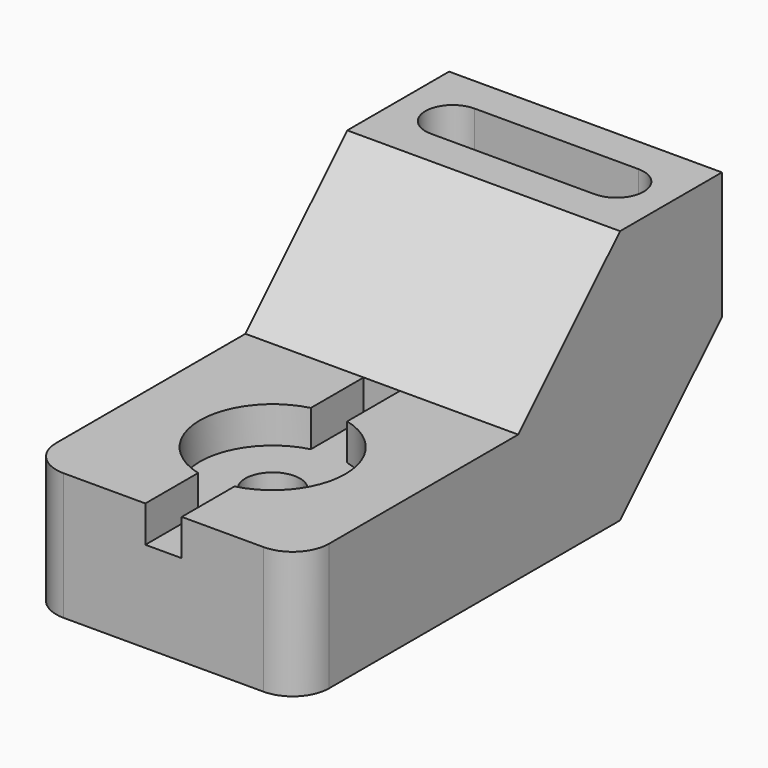
from build123d import *

# Parameters (mm, degrees)
F0_W           = 76.2
F0_H           = 35.56
F1_DEPTH       = 71.12
F0_H_2         = 76.2
F2_DEPTH       = 35.56
F4_DEPTH       = 76.2
F6_D           = 15.24
F6_CBORE_D     = 40.64
F6_CBORE_DEPTH = 10.16
F8_DEPTH       = 27.94
F10_DEPTH      = 10.16
F11_R          = 10.16


with BuildPart() as f1:
    # F0 (on Top) → F1 (new body)
    with BuildSketch(Plane.XY):
        with Locations((38.1, 129.54)):
            Rectangle(F0_W, F0_H)
        with Locations((38.1, 93.98)):
            Rectangle(F0_W, F0_H)
    extrude(amount=F1_DEPTH)

    # F0 (on Top) → F2 (join)
    with BuildSketch(Plane.XY):
        with Locations((38.1, 38.1)):
            Rectangle(F0_W, F0_H_2)
    extrude(amount=F2_DEPTH)

    # F3 (on face) → F4 (cut)
    with BuildSketch(Plane.YZ.offset(76.2)):
        Polygon((76.2, 71.12), (76.2, 35.56), (111.76, 71.12), align=None)
        Polygon((147.32, 0), (147.32, 35.56), (111.76, 0), align=None)
    extrude(amount=-F4_DEPTH, mode=Mode.SUBTRACT)

    # F6 (through all)
    with Locations(Plane.XY.offset(35.56)):
        with Locations((38.1, 38.1)):
            CounterBoreHole(F6_D / 2, F6_CBORE_D / 2, F6_CBORE_DEPTH)

    # F7 (on face) → F8 (cut)
    with BuildSketch(Plane.XY.offset(71.12)):
        with BuildLine():
            Line((60.96, 137.16), (15.24, 137.16))
            ThreePointArc((15.24, 137.16), (7.62, 129.54), (15.24, 121.92))
            Line((15.24, 121.92), (60.96, 121.92))
            ThreePointArc((60.96, 121.92), (68.58, 129.54), (60.96, 137.16))
        make_face()
    extrude(amount=-F8_DEPTH, mode=Mode.SUBTRACT)

    # F9 (on face) → F10 (cut)
    with BuildSketch(Plane.XY.offset(35.56)):
        with BuildLine():
            Line((43.18, 76.2), (33.02, 76.2))
            Line((33.02, 76.2), (33.02, 57.7747553987))
            ThreePointArc((33.02, 57.7747553987), (38.1, 58.42), (43.18, 57.7747553987))
            Line((43.18, 57.7747553987), (43.18, 76.2))
        make_face()
        with BuildLine():
            ThreePointArc((43.18, 18.4252446013), (38.1, 17.78), (33.02, 18.4252446013))
            Line((33.02, 18.4252446013), (33.02, 0))
            Line((33.02, 0), (43.18, 0))
            Line((43.18, 0), (43.18, 18.4252446013))
        make_face()
    extrude(amount=-F10_DEPTH, mode=Mode.SUBTRACT)

    # F11
    f11_edges = [f1.edges().sort_by_distance(p)[0] for p in [
        (76.2, 0, 17.78),
        (0, 0, 17.78),
    ]]
    fillet(f11_edges, radius=F11_R)


solid = f1.part
